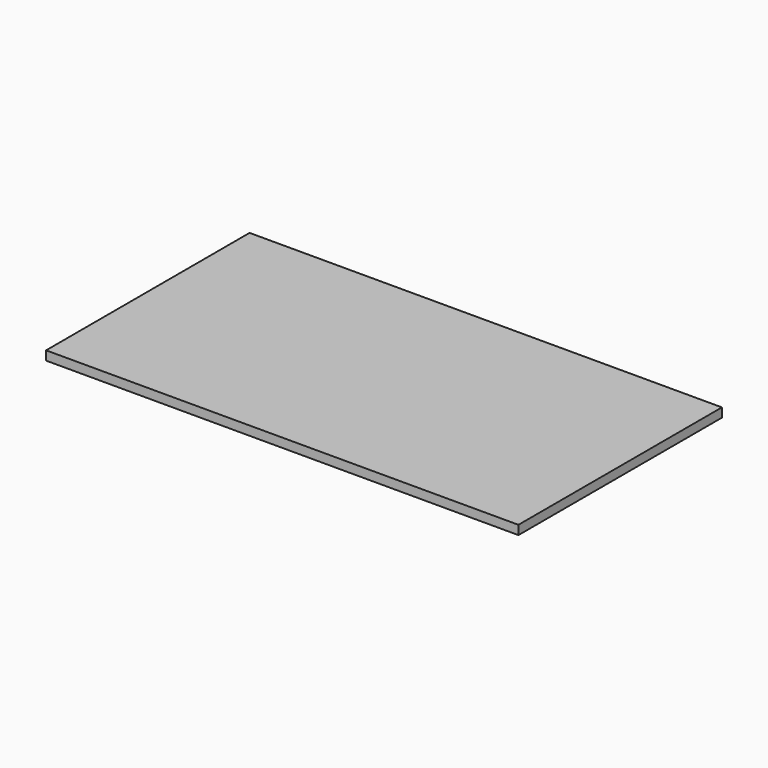
from build123d import *

# Parameters (mm, degrees)
F0_W     = 165.1
F0_H     = 88.9
F1_DEPTH = 3.175


# Not quite as in the source:
# - a length typed as a fraction of an inch, garbled in the dataset ("3 / 203.2 mm" for 3/8 in), is restored


with BuildPart() as f1:
    # F0 (on Top) → F1 (new body)
    with BuildSketch(Plane.XY):
        Rectangle(F0_W, F0_H)
    extrude(amount=F1_DEPTH)


solid = f1.part
